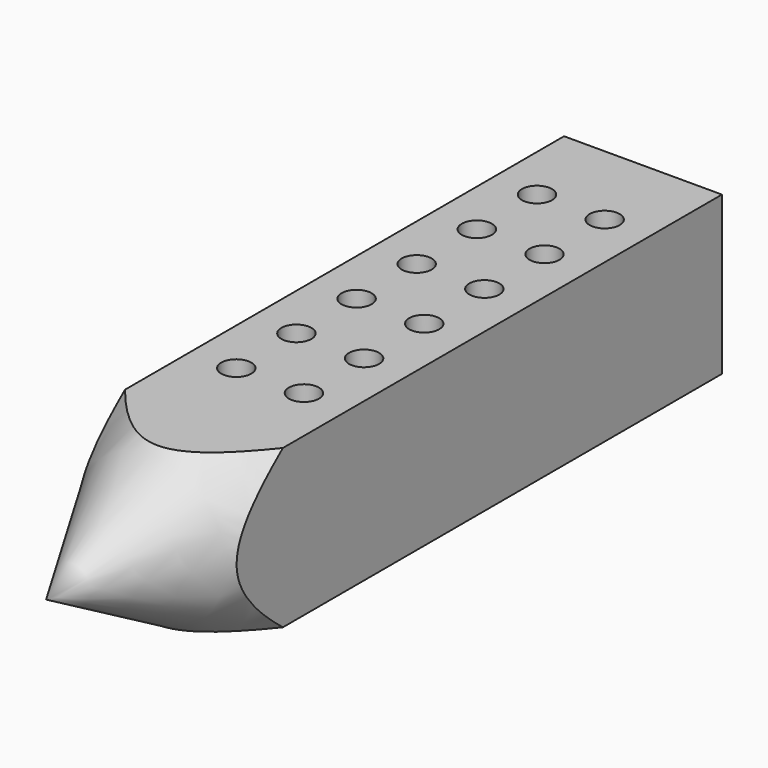
from build123d import *

# Parameters (mm, degrees)
F0_W      = 42
F0_H      = 42
F1_DEPTH  = 146
F2_R      = 29.6984848098
F4_R      = 21
F5_DEPTH  = 25
F6_R      = 21
F9_DEPTH  = 25
F7_R      = 21
F10_DEPTH = 25
F8_R      = 21
F11_DEPTH = 25
F12_R     = 4
F13_DEPTH = 20


# Not quite as in the source:
# - an extrude whose draft closes it to a point is written as a loft to that point


with BuildPart() as f1:
    # F0 (on Front) → F1 (new body)
    with BuildSketch(Plane.XZ):
        Rectangle(F0_W, F0_H)
    extrude(amount=F1_DEPTH)

    # F2 (on face) → F3 section 0
    with BuildSketch(Plane.XZ.offset(146), mode=Mode.PRIVATE) as f3_s0:
        Circle(F2_R)
    loft([f3_s0.sketch, Vertex(0, -198.4999999927, 0)], ruled=True)

    # F4 (on face) → F5 (cut)
    with BuildSketch(Plane(origin=(-21, 0, 0), x_dir=(0, -1, 0), z_dir=(-1, 0, 0))):
        with Locations((146, 0)):
            Circle(F4_R)
    extrude(amount=F5_DEPTH, mode=Mode.SUBTRACT)

    # F6 (on face) → F9 (cut)
    with BuildSketch(Plane.XY.offset(21)):
        with Locations((0, -146)):
            Circle(F6_R)
    extrude(amount=F9_DEPTH, mode=Mode.SUBTRACT)

    # F7 (on face) → F10 (cut)
    with BuildSketch(Plane.YZ.offset(21)):
        with Locations((-146, 0)):
            Circle(F7_R)
    extrude(amount=F10_DEPTH, mode=Mode.SUBTRACT)

    # F8 (on face) → F11 (cut)
    with BuildSketch(Plane(origin=(0, 0, -21), x_dir=(1, 0, 0), z_dir=(0, 0, -1))):
        with Locations((0, 146)):
            Circle(F8_R)
    extrude(amount=F11_DEPTH, mode=Mode.SUBTRACT)

    # F12 (on face) → F13 (cut)
    with BuildSketch(Plane.XY.offset(21)):
        with Locations((-9, -24)):
            Circle(F12_R)
        with Locations((-9, -44)):
            Circle(F12_R)
        with Locations((-9, -64)):
            Circle(F12_R)
        with Locations((-9, -84)):
            Circle(F12_R)
        with Locations((-9, -104)):
            Circle(F12_R)
        with Locations((-9, -124)):
            Circle(F12_R)
        with Locations((9, -24)):
            Circle(F12_R)
        with Locations((9, -44)):
            Circle(F12_R)
        with Locations((9, -64)):
            Circle(F12_R)
        with Locations((9, -84)):
            Circle(F12_R)
        with Locations((9, -104)):
            Circle(F12_R)
        with Locations((9, -124)):
            Circle(F12_R)
    extrude(amount=-F13_DEPTH, mode=Mode.SUBTRACT)


solid = f1.part
